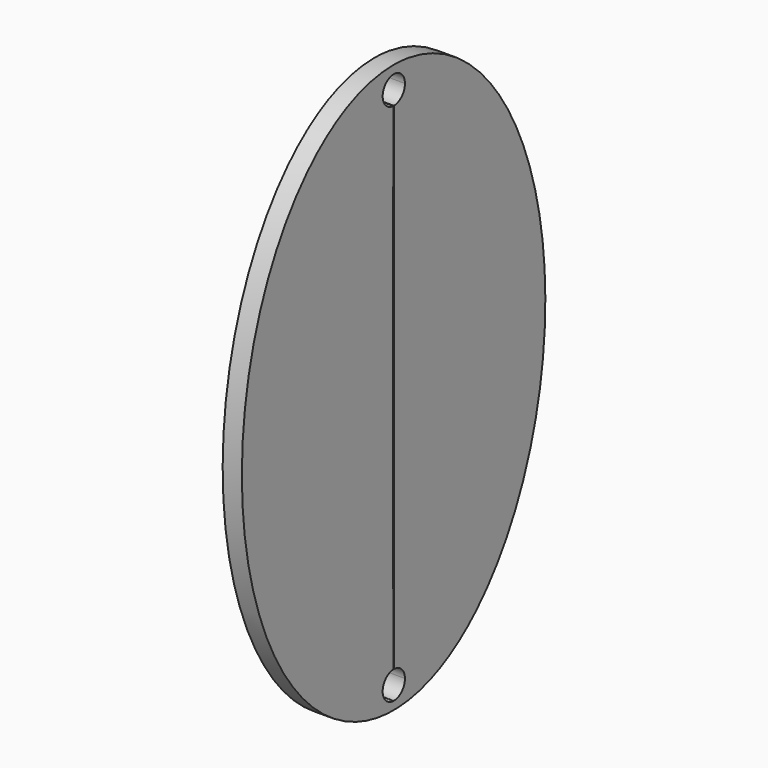
from build123d import *

# Parameters (mm, degrees)
F1_DEPTH = 5
F2_R     = 3.6307317185
F3_DEPTH = 5


# Not quite as in the source:
# - a pattern or mirror of a feature is missing from the dataset's text; its kind, count and spacing are read off the source's solid


with BuildPart() as f1:
    # F0 (on Right) → F1 (new body)
    with BuildSketch(Plane.YZ):
        with BuildLine():
            add(Edge.make_bspline(
                [(0, 74.0258097649), (-85.6036238732, 74.0258097649), (-42.8018119366, -37.0129048824), (0, -148.0516195297), (42.8018119366, -37.0129048824), (85.6036238732, 74.0258097649), (0, 74.0258097649)],
                knots=[0, 0, 0, 2.0943951024, 2.0943951024, 4.1887902048, 4.1887902048, 6.2831853072, 6.2831853072, 6.2831853072], degree=2, weights=[1, 0.5, 1, 0.5, 1, 0.5, 1]))
        make_face()
        with BuildLine():
            add(Edge.make_bspline(
                [(0, 72.9986578226), (-0.3155069903, 72.9986578226), (-0.1577534952, -36.4993289113), (0, -145.9973156452), (0.1577534952, -36.4993289113), (0.3155069903, 72.9986578226), (0, 72.9986578226)],
                knots=[0, 0, 0, 2.0943951024, 2.0943951024, 4.1887902048, 4.1887902048, 6.2831853072, 6.2831853072, 6.2831853072], degree=2, weights=[1, 0.5, 1, 0.5, 1, 0.5, 1]))
        make_face(mode=Mode.SUBTRACT)
    extrude(amount=F1_DEPTH)

    # F2 (on face) → F3 (cut)
    with BuildSketch(Plane.YZ.offset(5)):
        with Locations((0.0646514759, 68.2462112828)):
            Circle(F2_R)
    f3 = extrude(amount=-F3_DEPTH, mode=Mode.SUBTRACT)

    # F3_copies: F3 across plane
    add(f3.mirror(Plane(origin=(0, 0, 0), x_dir=(-1, 0, 0), z_dir=(0, 0, -1))), mode=Mode.SUBTRACT)


solid = f1.part
